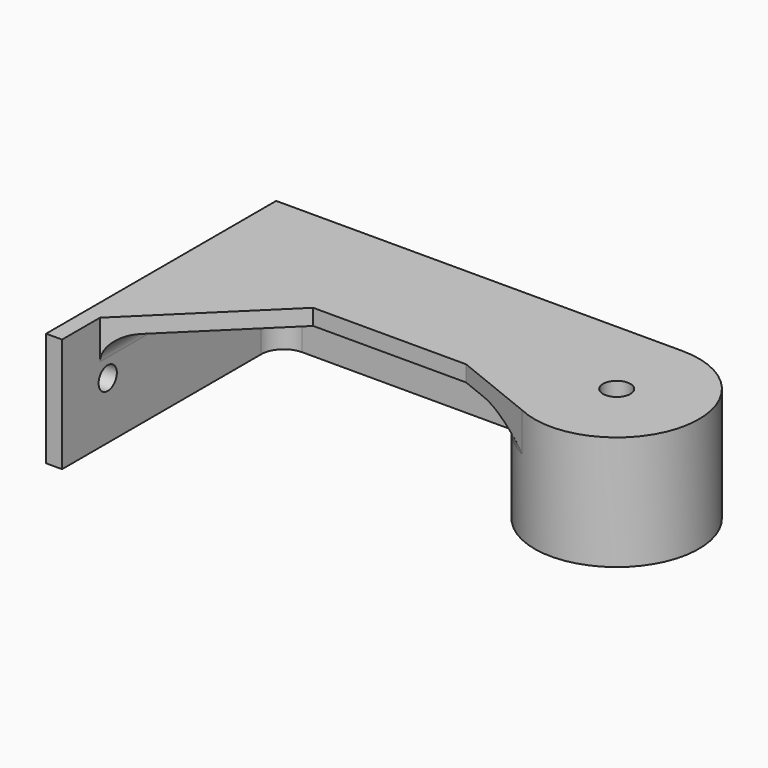
from build123d import *

# Parameters (mm, degrees)
F0_R      = 14.5
F1_DEPTH  = 25
F2_R      = 14.5
F3_DEPTH  = 3
F4_R      = 2.5
F5_DEPTH  = 25
F0_R_2    = 3
F6_DEPTH  = 30
F8_DEPTH  = 25
F9_DEPTH  = 3.5
F10_DEPTH = 30
F11_R     = 5


# Not quite as in the source:
# - a feature names something its author has since deleted; it is built from what else it names


with BuildPart() as f1:
    # F0 (on Top) → F1 (new body)
    with BuildSketch(Plane.XY):
        with BuildLine():
            Line((-44.2576195002, 24.5322410017), (-44.2576195002, -25.4677589983))
            Line((-44.2576195002, -25.4677589983), (-40.7576195002, -25.4677589983))
            Line((-40.7576195002, -25.4677589983), (-40.7576195002, 34.0321085225))
            Line((-40.7576195002, 34.0321085225), (26.7423804998, 34.0321085225))
            Line((26.7423804998, 34.0321085225), (26.7423804998, 19.5322410017))
            ThreePointArc((26.7423804998, 19.5322410017), (57.445862821, 6.7799260387), (44.8114401571, 37.5321085225))
            Line((44.8114401571, 37.5321085225), (44.6733208426, 37.5321085225))
            Line((44.6733208426, 37.5321085225), (-44.2576195002, 37.5321085225))
            Line((-44.2576195002, 37.5321085225), (-44.2576195002, 24.5322410017))
        make_face()
        with Locations((44.7423804998, 19.5322410017)):
            Circle(F0_R, mode=Mode.SUBTRACT)
    extrude(amount=F1_DEPTH)

    # F2 (on face) → F3 (join)
    with BuildSketch(Plane.XY.offset(25)):
        with BuildLine():
            ThreePointArc((26.7423804998, 19.5322410017), (29.5038185973, 9.9517279079), (36.9408506267, 3.3107696863))
            ThreePointArc((36.9408506267, 3.3107696863), (62.2844095115, 15.4977375434), (44.8114401571, 37.5321085225))
            Line((44.8114401571, 37.5321085225), (-44.2576195002, 37.5321085225))
            Line((-44.2576195002, 37.5321085225), (-44.2576195002, -25.4677589983))
            Line((-44.2576195002, -25.4677589983), (-40.7576195002, -25.4677589983))
            Line((-40.7576195002, -25.4677589983), (-40.7576195002, -15.0916781276))
            Line((-40.7576195002, -15.0916781276), (-40.7576195002, 34.0321085225))
            Line((-40.7576195002, 34.0321085225), (26.7423804998, 34.0321085225))
            Line((26.7423804998, 34.0321085225), (26.7423804998, 19.5322410017))
        make_face()
        with Locations((44.7423804998, 19.5322410017)):
            Circle(F2_R, mode=Mode.SUBTRACT)
    extrude(amount=-F3_DEPTH)

    # F4 (on face) → F5 (cut)
    with BuildSketch(Plane(origin=(-44.2576195002, 0, 0), x_dir=(0, -1, 0), z_dir=(-1, 0, 0))):
        with Locations((12.9677589983, 12.5)):
            Circle(F4_R)
    extrude(amount=-F5_DEPTH, mode=Mode.SUBTRACT)

    # F0 (on Top) → F6 (cut)
    with BuildSketch(Plane.XY):
        with Locations((44.7423804998, 19.5322410017)):
            Circle(F0_R_2)
    extrude(amount=F6_DEPTH, mode=Mode.SUBTRACT)

    # F4 (on face) → F8 (cut)
    with BuildSketch(Plane(origin=(-44.2576195002, 0, 0), x_dir=(0, -1, 0), z_dir=(-1, 0, 0))):
        with Locations((-22.0322410017, 12.5)):
            Circle(F4_R)
    extrude(amount=-F8_DEPTH, mode=Mode.SUBTRACT)

    # F2 (on face) → F9 (join)
    with BuildSketch(Plane.XY.offset(25)):
        with BuildLine():
            Line((18.9116307646, 10.5619383976), (36.9408506267, 3.3107696863))
            ThreePointArc((36.9408506267, 3.3107696863), (29.5038185973, 9.9517279079), (26.7423804998, 19.5322410017))
            Line((26.7423804998, 19.5322410017), (26.7423804998, 34.0321085225))
            Line((26.7423804998, 34.0321085225), (-40.7576195002, 34.0321085225))
            Line((-40.7576195002, 34.0321085225), (-40.7576195002, -15.0916781276))
            Line((-40.7576195002, -15.0916781276), (-14.5708816946, 10.5619383976))
            Line((-14.5708816946, 10.5619383976), (18.9116307646, 10.5619383976))
        make_face()
        with Locations((44.7423804998, 19.5322410017)):
            Circle(F2_R)
    extrude(amount=-F9_DEPTH)

    # F0 (on Top) → F10 (cut)
    with BuildSketch(Plane.XY):
        with Locations((44.7423804998, 19.5322410017)):
            Circle(F0_R_2)
    extrude(amount=F10_DEPTH, mode=Mode.SUBTRACT)

    # F11
    f11_edges = [f1.edges().sort_by_distance(p)[0] for p in [
        (26.74238, 34.032109, 10.75),
        (26.74238, 26.782175, 21.5),
        (-7.00762, 34.032109, 21.5),
        (-40.75762, 34.032109, 10.75),
        (-40.75762, 9.470215, 21.5),
    ]]
    fillet(f11_edges, radius=F11_R)


solid = f1.part
